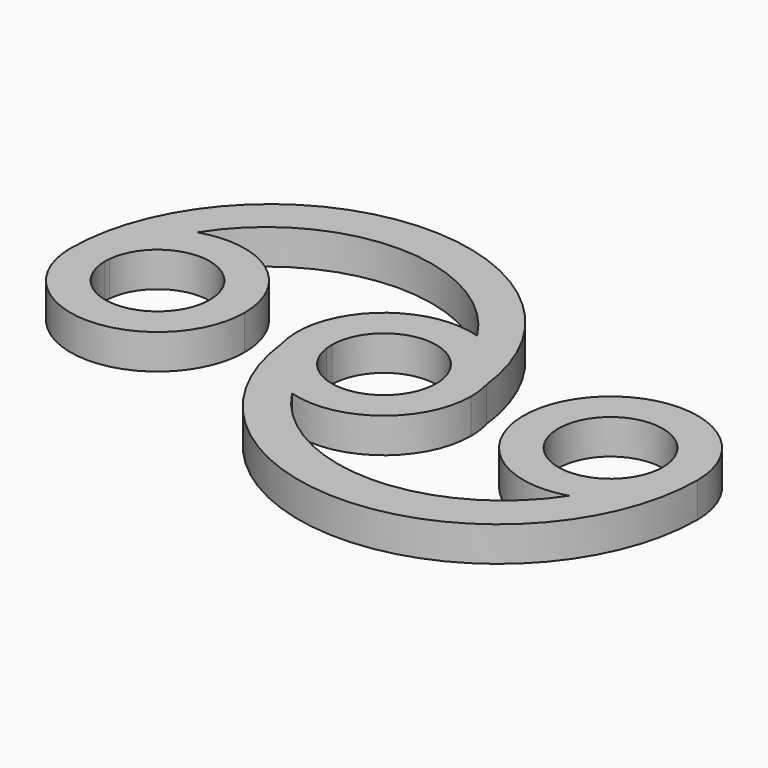
from build123d import *

# Parameters (mm, degrees)
F1_DEPTH = 5.08


# Not quite as in the source:
# - a feature names something its author has since deleted; it is built from what else it names


with BuildPart() as f1:
    # F0 (on Top) → F1 (new body)
    with BuildSketch(Plane.XY):
        with BuildLine():
            ThreePointArc((7.5830097901, 0.7499083436), (7.6107468293, 0.3754100423), (7.62, 0))
            ThreePointArc((7.62, 0), (0.4990141385, -7.6036428697), (-7.5546417033, -0.9958859045))
            ThreePointArc((-7.5546417033, -0.9958859045), (-6.3173271202, -6.8123022238), (-3.6964522326, -12.1501539452))
            ThreePointArc((-3.6964522326, -12.1501539452), (7.5612517696, -10.2037969245), (12.7, 0))
            ThreePointArc((12.7, 0), (12.5868786701, 1.6912969415), (12.249529867, 3.3524644721))
            ThreePointArc((12.249529867, 3.3524644721), (9.1791212991, 8.776886246), (3.897633179, 12.0871194088))
            ThreePointArc((3.897633179, 12.0871194088), (6.451051693, 6.6495502812), (7.5830097901, 0.7499083436))
        make_face()
        with BuildLine():
            ThreePointArc((-36.917633179, 12.0871194088), (-16.51, 23.3293611901), (3.897633179, 12.0871194088))
            ThreePointArc((3.897633179, 12.0871194088), (9.1791212991, 8.776886246), (12.249529867, 3.3524644721))
            ThreePointArc((12.249529867, 3.3524644721), (-18.3173290135, 29.0331939814), (-45.72, 0))
            ThreePointArc((-45.72, 0), (-43.286205272, 7.4762978347), (-36.917633179, 12.0871194088))
        make_face()
        with BuildLine():
            ThreePointArc((-20.32, 0), (-25.5437021653, 10.266205272), (-36.917633179, 12.0871194088))
            ThreePointArc((-36.917633179, 12.0871194088), (-43.286205272, 7.4762978347), (-45.72, 0))
            ThreePointArc((-45.72, 0), (-33.02, -12.7), (-20.32, 0))
        make_face()
        with BuildLine():
            ThreePointArc((-40.64, 0), (-40.6307468293, 0.3754100423), (-40.6030097901, 0.7499083436))
            ThreePointArc((-40.6030097901, 0.7499083436), (-32.6445899577, 7.6107468293), (-25.4, 0))
            ThreePointArc((-25.4, 0), (-33.02, -7.62), (-40.64, 0))
        make_face(mode=Mode.SUBTRACT)
        with BuildLine():
            ThreePointArc((36.7164522326, -12.1501539452), (16.51, -23.0707915841), (-3.6964522326, -12.1501539452))
            ThreePointArc((-3.6964522326, -12.1501539452), (-9.1059552655, -8.8527723739), (-12.249529867, -3.3524644721))
            ThreePointArc((-12.249529867, -3.3524644721), (18.3173290135, -29.0331939814), (45.72, 0))
            ThreePointArc((45.72, 0), (43.2237969245, -7.5612517696), (36.7164522326, -12.1501539452))
        make_face()
        with BuildLine():
            ThreePointArc((45.72, 0), (22.8162030755, 7.5612517696), (36.7164522326, -12.1501539452))
            ThreePointArc((36.7164522326, -12.1501539452), (43.2237969245, -7.5612517696), (45.72, 0))
        make_face()
        with BuildLine():
            ThreePointArc((40.64, 0), (40.6236428697, -0.4990141385), (40.5746417033, -0.9958859045))
            ThreePointArc((40.5746417033, -0.9958859045), (25.4163571303, 0.4990141385), (40.64, 0))
        make_face(mode=Mode.SUBTRACT)
        with BuildLine():
            ThreePointArc((-7.62, 0), (-0.3754100423, 7.6107468293), (7.5830097901, 0.7499083436))
            ThreePointArc((7.5830097901, 0.7499083436), (6.451051693, 6.6495502812), (3.897633179, 12.0871194088))
            ThreePointArc((3.897633179, 12.0871194088), (-8.776886246, 9.1791212991), (-12.249529867, -3.3524644721))
            ThreePointArc((-12.249529867, -3.3524644721), (-9.1059552655, -8.8527723739), (-3.6964522326, -12.1501539452))
            ThreePointArc((-3.6964522326, -12.1501539452), (-6.3173271202, -6.8123022238), (-7.5546417033, -0.9958859045))
            ThreePointArc((-7.5546417033, -0.9958859045), (-7.6036428697, -0.4990141385), (-7.62, 0))
        make_face()
    extrude(amount=F1_DEPTH)


solid = f1.part
